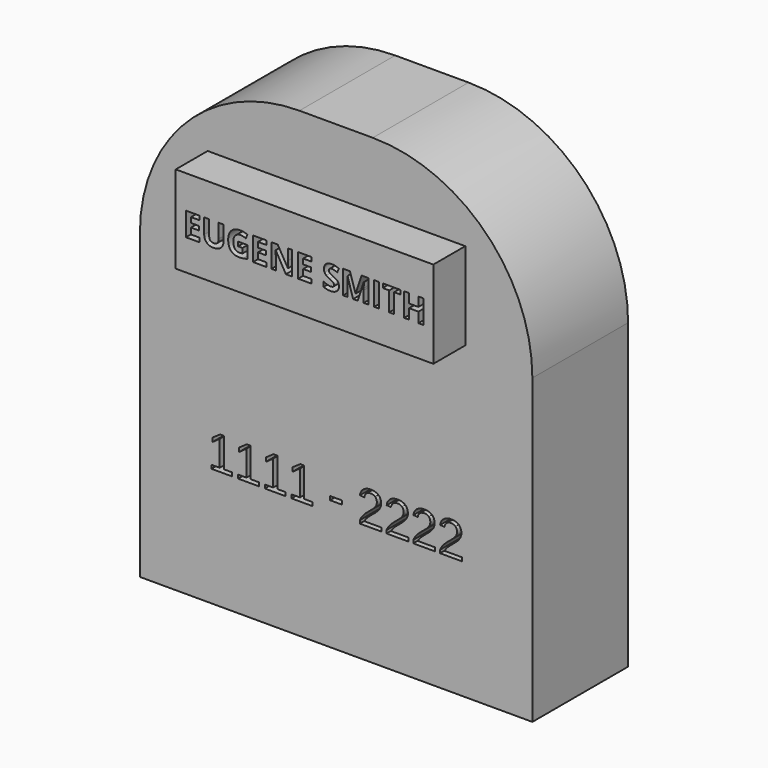
from build123d import *

# Parameters (mm, degrees)
F0_W     = 82.0154622197
F0_H     = 27.821501717
F0_W_2   = 1.5845067707
F0_H_2   = 7.4712192315
F1_DEPTH = 50.8
F0_W_3   = 3.7392849731
F0_H_3   = 1.1961884111
F2_DEPTH = 38.1


with BuildPart() as f1:
    # F0 (on Front) → F1 (new body)
    with BuildSketch(Plane.XZ):
        with Locations((-3.3327825367, 42.5519878045)):
            Rectangle(F0_W, F0_H)
        Polygon((-36.7796089812, 39.8028421267), (-36.7796089812, 38.4946838021), (-41.0818146713, 38.4946838021), (-41.0818146713, 45.9659030336), (-36.7796089812, 45.9659030336), (-36.7796089812, 44.6675558964), (-39.4973079006, 44.6675558964), (-39.4973079006, 43.0274523969), (-36.9676567404, 43.0274523969), (-36.9676567404, 41.7291052597), (-39.4973079006, 41.7291052597), (-39.4973079006, 39.8028421267), align=None, mode=Mode.SUBTRACT)
        with BuildLine():
            Line((-30.7195655424, 45.9659030336), (-29.1399643655, 45.9659030336))
            Line((-29.1399643655, 45.9659030336), (-29.1399643655, 41.1322580241))
            add(Edge.make_bspline(
                [(-29.1399643655, 41.1322580241), (-29.1399643655, 40.3032126859), (-29.5103366911, 39.6802022838)],
                knots=[0, 0, 0, 1, 1, 1], degree=2))
            add(Edge.make_bspline(
                [(-29.5103366911, 39.6802022838), (-29.8807090168, 39.0571918817), (-30.5813913194, 38.7244291079)],
                knots=[0, 0, 0, 1, 1, 1], degree=2))
            add(Edge.make_bspline(
                [(-30.5813913194, 38.7244291079), (-31.282073622, 38.3916663341), (-32.237029199, 38.3916663341)],
                knots=[0, 0, 0, 1, 1, 1], degree=2))
            add(Edge.make_bspline(
                [(-32.237029199, 38.3916663341), (-33.677638554, 38.3916663341), (-34.474797533, 39.1307757875)],
                knots=[0, 0, 0, 1, 1, 1], degree=2))
            add(Edge.make_bspline(
                [(-34.474797533, 39.1307757875), (-35.2719565121, 39.8698852409), (-35.2719565121, 41.151880399)],
                knots=[0, 0, 0, 1, 1, 1], degree=2))
            Line((-35.2719565121, 41.151880399), (-35.2719565121, 45.9659030336))
            Line((-35.2719565121, 45.9659030336), (-33.693990533, 45.9659030336))
            Line((-33.693990533, 45.9659030336), (-33.693990533, 41.3922544912))
            add(Edge.make_bspline(
                [(-33.693990533, 41.3922544912), (-33.693990533, 40.5288699969), (-33.3465109781, 40.1249761142)],
                knots=[0, 0, 0, 1, 1, 1], degree=2))
            add(Edge.make_bspline(
                [(-33.3465109781, 40.1249761142), (-32.9990314231, 39.7210822315), (-32.1961492513, 39.7210822315)],
                knots=[0, 0, 0, 1, 1, 1], degree=2))
            add(Edge.make_bspline(
                [(-32.1961492513, 39.7210822315), (-31.4194302461, 39.7210822315), (-31.0694978943, 40.127428911)],
                knots=[0, 0, 0, 1, 1, 1], degree=2))
            add(Edge.make_bspline(
                [(-31.0694978943, 40.127428911), (-30.7195655424, 40.5337755906), (-30.7195655424, 41.4020656786)],
                knots=[0, 0, 0, 1, 1, 1], degree=2))
            Line((-30.7195655424, 41.4020656786), (-30.7195655424, 45.9659030336))
        make_face(mode=Mode.SUBTRACT)
        with BuildLine():
            Line((-24.4747447403, 41.3709969184), (-24.4747447403, 42.6906016283))
            Line((-24.4747447403, 42.6906016283), (-21.5101309371, 42.6906016283))
            Line((-21.5101309371, 42.6906016283), (-21.5101309371, 38.8168177896))
            add(Edge.make_bspline(
                [(-21.5101309371, 38.8168177896), (-22.2312532136, 38.5813492911), (-22.8673451989, 38.4865078126)],
                knots=[0, 0, 0, 1, 1, 1], degree=2))
            add(Edge.make_bspline(
                [(-22.8673451989, 38.4865078126), (-23.5034371843, 38.3916663341), (-24.167327534, 38.3916663341)],
                knots=[0, 0, 0, 1, 1, 1], degree=2))
            add(Edge.make_bspline(
                [(-24.167327534, 38.3916663341), (-25.8581221686, 38.3916663341), (-26.7501226262, 39.3858666608)],
                knots=[0, 0, 0, 1, 1, 1], degree=2))
            add(Edge.make_bspline(
                [(-26.7501226262, 39.3858666608), (-27.6421230838, 40.3800669875), (-27.6421230838, 42.2409222043)],
                knots=[0, 0, 0, 1, 1, 1], degree=2))
            add(Edge.make_bspline(
                [(-27.6421230838, 42.2409222043), (-27.6421230838, 44.049451088), (-26.6070428094, 45.0608209928)],
                knots=[0, 0, 0, 1, 1, 1], degree=2))
            add(Edge.make_bspline(
                [(-26.6070428094, 45.0608209928), (-25.5719625351, 46.0721908975), (-23.7389056827, 46.0721908975)],
                knots=[0, 0, 0, 1, 1, 1], degree=2))
            add(Edge.make_bspline(
                [(-23.7389056827, 46.0721908975), (-22.587726357, 46.0721908975), (-21.5199421246, 45.612700286)],
                knots=[0, 0, 0, 1, 1, 1], degree=2))
            Line((-21.5199421246, 45.612700286), (-22.0464758502, 44.345421909))
            add(Edge.make_bspline(
                [(-22.0464758502, 44.345421909), (-22.8640748031, 44.7542213854), (-23.7487168701, 44.7542213854)],
                knots=[0, 0, 0, 1, 1, 1], degree=2))
            add(Edge.make_bspline(
                [(-23.7487168701, 44.7542213854), (-24.7756211549, 44.7542213854), (-25.3937259633, 44.0641678692)],
                knots=[0, 0, 0, 1, 1, 1], degree=2))
            add(Edge.make_bspline(
                [(-25.3937259633, 44.0641678692), (-26.0118307717, 43.374114353), (-26.0118307717, 42.209853444)],
                knots=[0, 0, 0, 1, 1, 1], degree=2))
            add(Edge.make_bspline(
                [(-26.0118307717, 42.209853444), (-26.0118307717, 40.9932662021), (-25.5139130094, 40.3522686231)],
                knots=[0, 0, 0, 1, 1, 1], degree=2))
            add(Edge.make_bspline(
                [(-25.5139130094, 40.3522686231), (-25.0159952471, 39.711271044), (-24.0659452638, 39.711271044)],
                knots=[0, 0, 0, 1, 1, 1], degree=2))
            add(Edge.make_bspline(
                [(-24.0659452638, 39.711271044), (-23.5688451005, 39.711271044), (-23.0586633539, 39.8126533142)],
                knots=[0, 0, 0, 1, 1, 1], degree=2))
            Line((-23.0586633539, 39.8126533142), (-23.0586633539, 41.3709969184))
            Line((-23.0586633539, 41.3709969184), (-24.4747447403, 41.3709969184))
        make_face(mode=Mode.SUBTRACT)
        Polygon((-15.4304651235, 39.8028421267), (-15.4304651235, 38.4946838021), (-19.7326708135, 38.4946838021), (-19.7326708135, 45.9659030336), (-15.4304651235, 45.9659030336), (-15.4304651235, 44.6675558964), (-18.1481640429, 44.6675558964), (-18.1481640429, 43.0274523969), (-15.6185128826, 43.0274523969), (-15.6185128826, 41.7291052597), (-18.1481640429, 41.7291052597), (-18.1481640429, 39.8028421267), align=None, mode=Mode.SUBTRACT)
        with BuildLine():
            Line((-7.2446644072, 45.9659030336), (-7.2446644072, 38.4946838021))
            Line((-7.2446644072, 38.4946838021), (-9.2575930292, 38.4946838021))
            Line((-9.2575930292, 38.4946838021), (-12.5083664658, 44.1459277645))
            Line((-12.5083664658, 44.1459277645), (-12.5541520072, 44.1459277645))
            add(Edge.make_bspline(
                [(-12.5541520072, 44.1459277645), (-12.4560401329, 42.6497216807), (-12.4560401329, 42.0103592995)],
                knots=[0, 0, 0, 1, 1, 1], degree=2))
            Line((-12.4560401329, 42.0103592995), (-12.4560401329, 38.4946838021))
            Line((-12.4560401329, 38.4946838021), (-13.8721215193, 38.4946838021))
            Line((-13.8721215193, 38.4946838021), (-13.8721215193, 45.9659030336))
            Line((-13.8721215193, 45.9659030336), (-11.8739096784, 45.9659030336))
            Line((-11.8739096784, 45.9659030336), (-8.6296770334, 40.3702558))
            Line((-8.6296770334, 40.3702558), (-8.5937026794, 40.3702558))
            add(Edge.make_bspline(
                [(-8.5937026794, 40.3702558), (-8.670556981, 41.8272171341), (-8.670556981, 42.4289699634)],
                knots=[0, 0, 0, 1, 1, 1], degree=2))
            Line((-8.670556981, 42.4289699634), (-8.670556981, 45.9659030336))
            Line((-8.670556981, 45.9659030336), (-7.2446644072, 45.9659030336))
        make_face(mode=Mode.SUBTRACT)
        Polygon((-1.0619811254, 39.8028421267), (-1.0619811254, 38.4946838021), (-5.3641868155, 38.4946838021), (-5.3641868155, 45.9659030336), (-1.0619811254, 45.9659030336), (-1.0619811254, 44.6675558964), (-3.7796800448, 44.6675558964), (-3.7796800448, 43.0274523969), (-1.2500288846, 43.0274523969), (-1.2500288846, 41.7291052597), (-3.7796800448, 41.7291052597), (-3.7796800448, 39.8028421267), align=None, mode=Mode.SUBTRACT)
        with BuildLine():
            add(Edge.make_bspline(
                [(7.2374658453, 41.8035067645), (7.6258253479, 41.3006834084), (7.6258253479, 40.5697499446)],
                knots=[0, 0, 0, 1, 1, 1], degree=2))
            add(Edge.make_bspline(
                [(7.6258253479, 40.5697499446), (7.6258253479, 39.5575624409), (6.8973446809, 38.9746143875)],
                knots=[0, 0, 0, 1, 1, 1], degree=2))
            add(Edge.make_bspline(
                [(6.8973446809, 38.9746143875), (6.1688640139, 38.3916663341), (4.8721520746, 38.3916663341)],
                knots=[0, 0, 0, 1, 1, 1], degree=2))
            add(Edge.make_bspline(
                [(4.8721520746, 38.3916663341), (3.6751872076, 38.3916663341), (2.7562059845, 38.8429809561)],
                knots=[0, 0, 0, 1, 1, 1], degree=2))
            Line((2.7562059845, 38.8429809561), (2.7562059845, 40.3146590713))
            add(Edge.make_bspline(
                [(2.7562059845, 40.3146590713), (3.511667417, 39.9761731048), (4.0357483458, 39.8388164807)],
                knots=[0, 0, 0, 1, 1, 1], degree=2))
            add(Edge.make_bspline(
                [(4.0357483458, 39.8388164807), (4.5598292746, 39.7014598566), (4.9947919175, 39.7014598566)],
                knots=[0, 0, 0, 1, 1, 1], degree=2))
            add(Edge.make_bspline(
                [(4.9947919175, 39.7014598566), (5.5147848516, 39.7014598566), (5.7935860945, 39.9001364021)],
                knots=[0, 0, 0, 1, 1, 1], degree=2))
            add(Edge.make_bspline(
                [(5.7935860945, 39.9001364021), (6.0723873374, 40.0988129477), (6.0723873374, 40.492895643)],
                knots=[0, 0, 0, 1, 1, 1], degree=2))
            add(Edge.make_bspline(
                [(6.0723873374, 40.492895643), (6.0723873374, 40.7120121624), (5.9497474945, 40.8837079425)],
                knots=[0, 0, 0, 1, 1, 1], degree=2))
            add(Edge.make_bspline(
                [(5.9497474945, 40.8837079425), (5.8271076516, 41.0554037226), (5.5891863563, 41.2132003205)],
                knots=[0, 0, 0, 1, 1, 1], degree=2))
            add(Edge.make_bspline(
                [(5.5891863563, 41.2132003205), (5.351265061, 41.3709969184), (4.6203315971, 41.7192940723)],
                knots=[0, 0, 0, 1, 1, 1], degree=2))
            add(Edge.make_bspline(
                [(4.6203315971, 41.7192940723), (3.9368188725, 42.0414280597), (3.5942449112, 42.3373988807)],
                knots=[0, 0, 0, 1, 1, 1], degree=2))
            add(Edge.make_bspline(
                [(3.5942449112, 42.3373988807), (3.25167095, 42.6333697016), (3.0472712118, 43.0274523969)],
                knots=[0, 0, 0, 1, 1, 1], degree=2))
            add(Edge.make_bspline(
                [(3.0472712118, 43.0274523969), (2.8428714735, 43.4215350922), (2.8428714735, 43.94643362)],
                knots=[0, 0, 0, 1, 1, 1], degree=2))
            add(Edge.make_bspline(
                [(2.8428714735, 43.94643362), (2.8428714735, 44.9389987488), (3.5149378128, 45.5055948231)],
                knots=[0, 0, 0, 1, 1, 1], degree=2))
            add(Edge.make_bspline(
                [(3.5149378128, 45.5055948231), (4.1870041521, 46.0721908975), (5.3725226338, 46.0721908975)],
                knots=[0, 0, 0, 1, 1, 1], degree=2))
            add(Edge.make_bspline(
                [(5.3725226338, 46.0721908975), (5.9546530882, 46.0721908975), (6.4836396107, 45.9348342734)],
                knots=[0, 0, 0, 1, 1, 1], degree=2))
            add(Edge.make_bspline(
                [(6.4836396107, 45.9348342734), (7.0126261333, 45.7974776493), (7.589850994, 45.5472923697)],
                knots=[0, 0, 0, 1, 1, 1], degree=2))
            Line((7.589850994, 45.5472923697), (7.0796692474, 44.3143531488))
            add(Edge.make_bspline(
                [(7.0796692474, 44.3143531488), (6.4811868139, 44.5596328346), (6.0903745144, 44.65692711)],
                knots=[0, 0, 0, 1, 1, 1], degree=2))
            add(Edge.make_bspline(
                [(6.0903745144, 44.65692711), (5.6995622149, 44.7542213854), (5.3218314987, 44.7542213854)],
                knots=[0, 0, 0, 1, 1, 1], degree=2))
            add(Edge.make_bspline(
                [(5.3218314987, 44.7542213854), (4.8721520746, 44.7542213854), (4.6317779825, 44.5449160535)],
                knots=[0, 0, 0, 1, 1, 1], degree=2))
            add(Edge.make_bspline(
                [(4.6317779825, 44.5449160535), (4.3914038903, 44.3356107215), (4.3914038903, 43.998759953)],
                knots=[0, 0, 0, 1, 1, 1], degree=2))
            add(Edge.make_bspline(
                [(4.3914038903, 43.998759953), (4.3914038903, 43.789454621), (4.4886981657, 43.633293221)],
                knots=[0, 0, 0, 1, 1, 1], degree=2))
            add(Edge.make_bspline(
                [(4.4886981657, 43.633293221), (4.5859924411, 43.477131821), (4.7977505699, 43.3315992074)],
                knots=[0, 0, 0, 1, 1, 1], degree=2))
            add(Edge.make_bspline(
                [(4.7977505699, 43.3315992074), (5.0095086987, 43.1860665938), (5.8009444851, 42.8083358776)],
                knots=[0, 0, 0, 1, 1, 1], degree=2))
            add(Edge.make_bspline(
                [(5.8009444851, 42.8083358776), (6.8491063427, 42.3063301205), (7.2374658453, 41.8035067645)],
                knots=[0, 0, 0, 1, 1, 1], degree=2))
        make_face(mode=Mode.SUBTRACT)
        with BuildLine():
            Line((13.594297704, 38.4946838021), (12.1422419637, 38.4946838021))
            Line((12.1422419637, 38.4946838021), (10.3435242673, 44.3552330964))
            Line((10.3435242673, 44.3552330964), (10.297738726, 44.3552330964))
            add(Edge.make_bspline(
                [(10.297738726, 44.3552330964), (10.3958506003, 42.5679617854), (10.3958506003, 41.9694793519)],
                knots=[0, 0, 0, 1, 1, 1], degree=2))
            Line((10.3958506003, 41.9694793519), (10.3958506003, 38.4946838021))
            Line((10.3958506003, 38.4946838021), (8.9797692139, 38.4946838021))
            Line((8.9797692139, 38.4946838021), (8.9797692139, 45.9659030336))
            Line((8.9797692139, 45.9659030336), (11.1365952516, 45.9659030336))
            Line((11.1365952516, 45.9659030336), (12.9042441878, 40.2525215508))
            Line((12.9042441878, 40.2525215508), (12.935312948, 40.2525215508))
            Line((12.935312948, 40.2525215508), (14.8108849459, 45.9659030336))
            Line((14.8108849459, 45.9659030336), (16.9660757857, 45.9659030336))
            Line((16.9660757857, 45.9659030336), (16.9660757857, 38.4946838021))
            Line((16.9660757857, 38.4946838021), (15.4894920768, 38.4946838021))
            Line((15.4894920768, 38.4946838021), (15.4894920768, 42.0316168723))
            add(Edge.make_bspline(
                [(15.4894920768, 42.0316168723), (15.4894920768, 42.2818021519), (15.4976680663, 42.608841733)],
                knots=[0, 0, 0, 1, 1, 1], degree=2))
            add(Edge.make_bspline(
                [(15.4976680663, 42.608841733), (15.5058440558, 42.9358813142), (15.5663463783, 44.345421909)],
                knots=[0, 0, 0, 1, 1, 1], degree=2))
            Line((15.5663463783, 44.345421909), (15.520560837, 44.345421909))
            Line((15.520560837, 44.345421909), (13.594297704, 38.4946838021))
        make_face(mode=Mode.SUBTRACT)
        with Locations((19.6388067627, 42.2302934179)):
            Rectangle(F0_W_2, F0_H_2, mode=Mode.SUBTRACT)
        Polygon((25.1943916475, 44.6479335215), (25.1943916475, 38.4946838021), (23.6098848768, 38.4946838021), (23.6098848768, 44.6479335215), (21.5806042758, 44.6479335215), (21.5806042758, 45.9659030336), (27.2220370507, 45.9659030336), (27.2220370507, 44.6479335215), align=None, mode=Mode.SUBTRACT)
        Polygon((34.4937621377, 45.9659030336), (34.4937621377, 38.4946838021), (32.9141609607, 38.4946838021), (32.9141609607, 41.7192940723), (29.9560879491, 41.7192940723), (29.9560879491, 38.4946838021), (28.3715811784, 38.4946838021), (28.3715811784, 45.9659030336), (29.9560879491, 45.9659030336), (29.9560879491, 43.0372635844), (32.9141609607, 43.0372635844), (32.9141609607, 45.9659030336), align=None, mode=Mode.SUBTRACT)
    extrude(amount=F1_DEPTH)

    # F0 (on Front) → F2 (join)
    with BuildSketch(Plane.XZ):
        with BuildLine():
            Line((-65.9075155854, 26.4598572791), (-65.9075155854, -69.9368044734))
            Line((-65.9075155854, -69.9368044734), (59.0424365504, -69.9368044734))
            Line((59.0424365504, -69.9368044734), (59.0424365504, 26.4598572791))
            ThreePointArc((59.0424365504, 26.4598572791), (44.1634610346, 62.3808817633), (8.2424365504, 77.2598572791))
            Line((8.2424365504, 77.2598572791), (-15.1075155854, 77.2598572791))
            ThreePointArc((-15.1075155854, 77.2598572791), (-51.0285400697, 62.3808817633), (-65.9075155854, 26.4598572791))
        make_face()
        Polygon((-36.5724661048, -32.2220926494), (-43.1730337574, -32.2220926494), (-43.1730337574, -31.0785365283), (-40.4911793396, -31.0785365283), (-40.4911793396, -22.9731638546), (-42.8668095241, -24.6717513984), (-42.8668095241, -23.399006929), (-40.378737629, -21.6884575011), (-39.1370940583, -21.6884575011), (-39.1370940583, -31.0785365283), (-36.5724661048, -31.0785365283), align=None, mode=Mode.SUBTRACT)
        Polygon((-28.0579969945, -32.2220926494), (-34.658564647, -32.2220926494), (-34.658564647, -31.0785365283), (-31.9767102293, -31.0785365283), (-31.9767102293, -22.9731638546), (-34.3523404138, -24.6717513984), (-34.3523404138, -23.399006929), (-31.8642685187, -21.6884575011), (-30.6226249479, -21.6884575011), (-30.6226249479, -31.0785365283), (-28.0579969945, -31.0785365283), align=None, mode=Mode.SUBTRACT)
        Polygon((-19.5435278842, -32.2220926494), (-26.1440955367, -32.2220926494), (-26.1440955367, -31.0785365283), (-23.462241119, -31.0785365283), (-23.462241119, -22.9731638546), (-25.8378713035, -24.6717513984), (-25.8378713035, -23.399006929), (-23.3497994083, -21.6884575011), (-22.1081558376, -21.6884575011), (-22.1081558376, -31.0785365283), (-19.5435278842, -31.0785365283), align=None, mode=Mode.SUBTRACT)
        Polygon((-11.0290587739, -32.2220926494), (-17.6296264264, -32.2220926494), (-17.6296264264, -31.0785365283), (-14.9477720087, -31.0785365283), (-14.9477720087, -22.9731638546), (-17.3234021932, -24.6717513984), (-17.3234021932, -23.399006929), (-14.835330298, -21.6884575011), (-13.5936867273, -21.6884575011), (-13.5936867273, -31.0785365283), (-11.0290587739, -31.0785365283), align=None, mode=Mode.SUBTRACT)
        with Locations((-3.4799137113, -28.1550520516)):
            Rectangle(F0_W_3, F0_H_3, mode=Mode.SUBTRACT)
        with BuildLine():
            Line((11.0693259331, -32.2220926494), (4.0931551195, -32.2220926494))
            Line((4.0931551195, -32.2220926494), (4.0931551195, -31.2723190509))
            add(Edge.make_bspline(
                [(4.0931551195, -31.2723190509), (4.4735430342, -30.396709134), (5.0237897033, -29.7280398122)],
                knots=[0, 0, 0, 1, 1, 1], degree=2))
            add(Edge.make_bspline(
                [(5.0237897033, -29.7280398122), (5.5740363724, -29.0593704904), (6.1793077084, -28.5174971401)],
                knots=[0, 0, 0, 1, 1, 1], degree=2))
            add(Edge.make_bspline(
                [(6.1793077084, -28.5174971401), (6.7845790445, -27.9756237899), (7.3790846848, -27.5115026864)],
                knots=[0, 0, 0, 1, 1, 1], degree=2))
            add(Edge.make_bspline(
                [(7.3790846848, -27.5115026864), (7.9735903251, -27.0473815829), (8.4520656896, -26.5844566678)],
                knots=[0, 0, 0, 1, 1, 1], degree=2))
            add(Edge.make_bspline(
                [(8.4520656896, -26.5844566678), (8.930541054, -26.1215317527), (9.2259995916, -25.613151678)],
                knots=[0, 0, 0, 1, 1, 1], degree=2))
            add(Edge.make_bspline(
                [(9.2259995916, -25.613151678), (9.5214581291, -25.1047716032), (9.5214581291, -24.4612222381)],
                knots=[0, 0, 0, 1, 1, 1], degree=2))
            add(Edge.make_bspline(
                [(9.5214581291, -24.4612222381), (9.5214581291, -23.5951818284), (9.0130780544, -23.116706464)],
                knots=[0, 0, 0, 1, 1, 1], degree=2))
            add(Edge.make_bspline(
                [(9.0130780544, -23.116706464), (8.5046979797, -22.6382310995), (7.6003795408, -22.6382310995)],
                knots=[0, 0, 0, 1, 1, 1], degree=2))
            add(Edge.make_bspline(
                [(7.6003795408, -22.6382310995), (6.7391238848, -22.6382310995), (6.1828962737, -23.1047445798)],
                knots=[0, 0, 0, 1, 1, 1], degree=2))
            add(Edge.make_bspline(
                [(6.1828962737, -23.1047445798), (5.6266686625, -23.5712580602), (5.5285812128, -24.4157670784)],
                knots=[0, 0, 0, 1, 1, 1], degree=2))
            Line((5.5285812128, -24.4157670784), (4.15296454, -24.2889711069))
            add(Edge.make_bspline(
                [(4.15296454, -24.2889711069), (4.301291903, -23.0257961447), (5.2247493564, -22.2781783878)],
                knots=[0, 0, 0, 1, 1, 1], degree=2))
            add(Edge.make_bspline(
                [(5.2247493564, -22.2781783878), (6.1482068098, -21.5305606308), (7.6003795408, -21.5305606308)],
                knots=[0, 0, 0, 1, 1, 1], degree=2))
            add(Edge.make_bspline(
                [(7.6003795408, -21.5305606308), (9.1913101276, -21.5305606308), (10.04778103, -22.281766953)],
                knots=[0, 0, 0, 1, 1, 1], degree=2))
            add(Edge.make_bspline(
                [(10.04778103, -22.281766953), (10.9042519324, -23.0329732752), (10.9042519324, -24.4157670784)],
                knots=[0, 0, 0, 1, 1, 1], degree=2))
            add(Edge.make_bspline(
                [(10.9042519324, -24.4157670784), (10.9042519324, -25.0306079217), (10.6231476557, -25.6358792578)],
                knots=[0, 0, 0, 1, 1, 1], degree=2))
            add(Edge.make_bspline(
                [(10.6231476557, -25.6358792578), (10.3420433791, -26.2411505938), (9.7894043332, -26.8464219298)],
                knots=[0, 0, 0, 1, 1, 1], degree=2))
            add(Edge.make_bspline(
                [(9.7894043332, -26.8464219298), (9.2367652873, -27.4516932658), (7.6745432223, -28.7220453584)],
                knots=[0, 0, 0, 1, 1, 1], degree=2))
            add(Edge.make_bspline(
                [(7.6745432223, -28.7220453584), (6.8132875663, -29.4254041442), (6.3049074916, -29.9900050742)],
                knots=[0, 0, 0, 1, 1, 1], degree=2))
            add(Edge.make_bspline(
                [(6.3049074916, -29.9900050742), (5.7965274169, -30.5546060043), (5.5740363724, -31.0785365283)],
                knots=[0, 0, 0, 1, 1, 1], degree=2))
            Line((5.5740363724, -31.0785365283), (11.0693259331, -31.0785365283))
            Line((11.0693259331, -31.0785365283), (11.0693259331, -32.2220926494))
        make_face(mode=Mode.SUBTRACT)
        with BuildLine():
            Line((19.5837950434, -32.2220926494), (12.6076242298, -32.2220926494))
            Line((12.6076242298, -32.2220926494), (12.6076242298, -31.2723190509))
            add(Edge.make_bspline(
                [(12.6076242298, -31.2723190509), (12.9880121445, -30.396709134), (13.5382588136, -29.7280398122)],
                knots=[0, 0, 0, 1, 1, 1], degree=2))
            add(Edge.make_bspline(
                [(13.5382588136, -29.7280398122), (14.0885054827, -29.0593704904), (14.6937768188, -28.5174971401)],
                knots=[0, 0, 0, 1, 1, 1], degree=2))
            add(Edge.make_bspline(
                [(14.6937768188, -28.5174971401), (15.2990481548, -27.9756237899), (15.8935537951, -27.5115026864)],
                knots=[0, 0, 0, 1, 1, 1], degree=2))
            add(Edge.make_bspline(
                [(15.8935537951, -27.5115026864), (16.4880594354, -27.0473815829), (16.9665347999, -26.5844566678)],
                knots=[0, 0, 0, 1, 1, 1], degree=2))
            add(Edge.make_bspline(
                [(16.9665347999, -26.5844566678), (17.4450101643, -26.1215317527), (17.7404687019, -25.613151678)],
                knots=[0, 0, 0, 1, 1, 1], degree=2))
            add(Edge.make_bspline(
                [(17.7404687019, -25.613151678), (18.0359272394, -25.1047716032), (18.0359272394, -24.4612222381)],
                knots=[0, 0, 0, 1, 1, 1], degree=2))
            add(Edge.make_bspline(
                [(18.0359272394, -24.4612222381), (18.0359272394, -23.5951818284), (17.5275471647, -23.116706464)],
                knots=[0, 0, 0, 1, 1, 1], degree=2))
            add(Edge.make_bspline(
                [(17.5275471647, -23.116706464), (17.01916709, -22.6382310995), (16.1148486512, -22.6382310995)],
                knots=[0, 0, 0, 1, 1, 1], degree=2))
            add(Edge.make_bspline(
                [(16.1148486512, -22.6382310995), (15.2535929952, -22.6382310995), (14.697365384, -23.1047445798)],
                knots=[0, 0, 0, 1, 1, 1], degree=2))
            add(Edge.make_bspline(
                [(14.697365384, -23.1047445798), (14.1411377728, -23.5712580602), (14.0430503231, -24.4157670784)],
                knots=[0, 0, 0, 1, 1, 1], degree=2))
            Line((14.0430503231, -24.4157670784), (12.6674336503, -24.2889711069))
            add(Edge.make_bspline(
                [(12.6674336503, -24.2889711069), (12.8157610133, -23.0257961447), (13.7392184667, -22.2781783878)],
                knots=[0, 0, 0, 1, 1, 1], degree=2))
            add(Edge.make_bspline(
                [(13.7392184667, -22.2781783878), (14.6626759201, -21.5305606308), (16.1148486512, -21.5305606308)],
                knots=[0, 0, 0, 1, 1, 1], degree=2))
            add(Edge.make_bspline(
                [(16.1148486512, -21.5305606308), (17.705779238, -21.5305606308), (18.5622501403, -22.281766953)],
                knots=[0, 0, 0, 1, 1, 1], degree=2))
            add(Edge.make_bspline(
                [(18.5622501403, -22.281766953), (19.4187210427, -23.0329732752), (19.4187210427, -24.4157670784)],
                knots=[0, 0, 0, 1, 1, 1], degree=2))
            add(Edge.make_bspline(
                [(19.4187210427, -24.4157670784), (19.4187210427, -25.0306079217), (19.1376167661, -25.6358792578)],
                knots=[0, 0, 0, 1, 1, 1], degree=2))
            add(Edge.make_bspline(
                [(19.1376167661, -25.6358792578), (18.8565124894, -26.2411505938), (18.3038734435, -26.8464219298)],
                knots=[0, 0, 0, 1, 1, 1], degree=2))
            add(Edge.make_bspline(
                [(18.3038734435, -26.8464219298), (17.7512343976, -27.4516932658), (16.1890123327, -28.7220453584)],
                knots=[0, 0, 0, 1, 1, 1], degree=2))
            add(Edge.make_bspline(
                [(16.1890123327, -28.7220453584), (15.3277566767, -29.4254041442), (14.8193766019, -29.9900050742)],
                knots=[0, 0, 0, 1, 1, 1], degree=2))
            add(Edge.make_bspline(
                [(14.8193766019, -29.9900050742), (14.3109965272, -30.5546060043), (14.0885054827, -31.0785365283)],
                knots=[0, 0, 0, 1, 1, 1], degree=2))
            Line((14.0885054827, -31.0785365283), (19.5837950434, -31.0785365283))
            Line((19.5837950434, -31.0785365283), (19.5837950434, -32.2220926494))
        make_face(mode=Mode.SUBTRACT)
        with BuildLine():
            Line((28.0982641537, -32.2220926494), (21.1220933401, -32.2220926494))
            Line((21.1220933401, -32.2220926494), (21.1220933401, -31.2723190509))
            add(Edge.make_bspline(
                [(21.1220933401, -31.2723190509), (21.5024812548, -30.396709134), (22.0527279239, -29.7280398122)],
                knots=[0, 0, 0, 1, 1, 1], degree=2))
            add(Edge.make_bspline(
                [(22.0527279239, -29.7280398122), (22.6029745931, -29.0593704904), (23.2082459291, -28.5174971401)],
                knots=[0, 0, 0, 1, 1, 1], degree=2))
            add(Edge.make_bspline(
                [(23.2082459291, -28.5174971401), (23.8135172651, -27.9756237899), (24.4080229054, -27.5115026864)],
                knots=[0, 0, 0, 1, 1, 1], degree=2))
            add(Edge.make_bspline(
                [(24.4080229054, -27.5115026864), (25.0025285458, -27.0473815829), (25.4810039102, -26.5844566678)],
                knots=[0, 0, 0, 1, 1, 1], degree=2))
            add(Edge.make_bspline(
                [(25.4810039102, -26.5844566678), (25.9594792746, -26.1215317527), (26.2549378122, -25.613151678)],
                knots=[0, 0, 0, 1, 1, 1], degree=2))
            add(Edge.make_bspline(
                [(26.2549378122, -25.613151678), (26.5503963497, -25.1047716032), (26.5503963497, -24.4612222381)],
                knots=[0, 0, 0, 1, 1, 1], degree=2))
            add(Edge.make_bspline(
                [(26.5503963497, -24.4612222381), (26.5503963497, -23.5951818284), (26.042016275, -23.116706464)],
                knots=[0, 0, 0, 1, 1, 1], degree=2))
            add(Edge.make_bspline(
                [(26.042016275, -23.116706464), (25.5336362003, -22.6382310995), (24.6293177615, -22.6382310995)],
                knots=[0, 0, 0, 1, 1, 1], degree=2))
            add(Edge.make_bspline(
                [(24.6293177615, -22.6382310995), (23.7680621055, -22.6382310995), (23.2118344943, -23.1047445798)],
                knots=[0, 0, 0, 1, 1, 1], degree=2))
            add(Edge.make_bspline(
                [(23.2118344943, -23.1047445798), (22.6556068831, -23.5712580602), (22.5575194334, -24.4157670784)],
                knots=[0, 0, 0, 1, 1, 1], degree=2))
            Line((22.5575194334, -24.4157670784), (21.1819027607, -24.2889711069))
            add(Edge.make_bspline(
                [(21.1819027607, -24.2889711069), (21.3302301236, -23.0257961447), (22.253687577, -22.2781783878)],
                knots=[0, 0, 0, 1, 1, 1], degree=2))
            add(Edge.make_bspline(
                [(22.253687577, -22.2781783878), (23.1771450304, -21.5305606308), (24.6293177615, -21.5305606308)],
                knots=[0, 0, 0, 1, 1, 1], degree=2))
            add(Edge.make_bspline(
                [(24.6293177615, -21.5305606308), (26.2202483483, -21.5305606308), (27.0767192506, -22.281766953)],
                knots=[0, 0, 0, 1, 1, 1], degree=2))
            add(Edge.make_bspline(
                [(27.0767192506, -22.281766953), (27.933190153, -23.0329732752), (27.933190153, -24.4157670784)],
                knots=[0, 0, 0, 1, 1, 1], degree=2))
            add(Edge.make_bspline(
                [(27.933190153, -24.4157670784), (27.933190153, -25.0306079217), (27.6520858764, -25.6358792578)],
                knots=[0, 0, 0, 1, 1, 1], degree=2))
            add(Edge.make_bspline(
                [(27.6520858764, -25.6358792578), (27.3709815998, -26.2411505938), (26.8183425538, -26.8464219298)],
                knots=[0, 0, 0, 1, 1, 1], degree=2))
            add(Edge.make_bspline(
                [(26.8183425538, -26.8464219298), (26.2657035079, -27.4516932658), (24.703481443, -28.7220453584)],
                knots=[0, 0, 0, 1, 1, 1], degree=2))
            add(Edge.make_bspline(
                [(24.703481443, -28.7220453584), (23.842225787, -29.4254041442), (23.3338457123, -29.9900050742)],
                knots=[0, 0, 0, 1, 1, 1], degree=2))
            add(Edge.make_bspline(
                [(23.3338457123, -29.9900050742), (22.8254656375, -30.5546060043), (22.6029745931, -31.0785365283)],
                knots=[0, 0, 0, 1, 1, 1], degree=2))
            Line((22.6029745931, -31.0785365283), (28.0982641537, -31.0785365283))
            Line((28.0982641537, -31.0785365283), (28.0982641537, -32.2220926494))
        make_face(mode=Mode.SUBTRACT)
        with BuildLine():
            Line((36.612733264, -32.2220926494), (29.6365624504, -32.2220926494))
            Line((29.6365624504, -32.2220926494), (29.6365624504, -31.2723190509))
            add(Edge.make_bspline(
                [(29.6365624504, -31.2723190509), (30.0169503652, -30.396709134), (30.5671970343, -29.7280398122)],
                knots=[0, 0, 0, 1, 1, 1], degree=2))
            add(Edge.make_bspline(
                [(30.5671970343, -29.7280398122), (31.1174437034, -29.0593704904), (31.7227150394, -28.5174971401)],
                knots=[0, 0, 0, 1, 1, 1], degree=2))
            add(Edge.make_bspline(
                [(31.7227150394, -28.5174971401), (32.3279863754, -27.9756237899), (32.9224920158, -27.5115026864)],
                knots=[0, 0, 0, 1, 1, 1], degree=2))
            add(Edge.make_bspline(
                [(32.9224920158, -27.5115026864), (33.5169976561, -27.0473815829), (33.9954730205, -26.5844566678)],
                knots=[0, 0, 0, 1, 1, 1], degree=2))
            add(Edge.make_bspline(
                [(33.9954730205, -26.5844566678), (34.473948385, -26.1215317527), (34.7694069225, -25.613151678)],
                knots=[0, 0, 0, 1, 1, 1], degree=2))
            add(Edge.make_bspline(
                [(34.7694069225, -25.613151678), (35.0648654601, -25.1047716032), (35.0648654601, -24.4612222381)],
                knots=[0, 0, 0, 1, 1, 1], degree=2))
            add(Edge.make_bspline(
                [(35.0648654601, -24.4612222381), (35.0648654601, -23.5951818284), (34.5564853853, -23.116706464)],
                knots=[0, 0, 0, 1, 1, 1], degree=2))
            add(Edge.make_bspline(
                [(34.5564853853, -23.116706464), (34.0481053106, -22.6382310995), (33.1437868718, -22.6382310995)],
                knots=[0, 0, 0, 1, 1, 1], degree=2))
            add(Edge.make_bspline(
                [(33.1437868718, -22.6382310995), (32.2825312158, -22.6382310995), (31.7263036046, -23.1047445798)],
                knots=[0, 0, 0, 1, 1, 1], degree=2))
            add(Edge.make_bspline(
                [(31.7263036046, -23.1047445798), (31.1700759935, -23.5712580602), (31.0719885438, -24.4157670784)],
                knots=[0, 0, 0, 1, 1, 1], degree=2))
            Line((31.0719885438, -24.4157670784), (29.696371871, -24.2889711069))
            add(Edge.make_bspline(
                [(29.696371871, -24.2889711069), (29.844699234, -23.0257961447), (30.7681566873, -22.2781783878)],
                knots=[0, 0, 0, 1, 1, 1], degree=2))
            add(Edge.make_bspline(
                [(30.7681566873, -22.2781783878), (31.6916141407, -21.5305606308), (33.1437868718, -21.5305606308)],
                knots=[0, 0, 0, 1, 1, 1], degree=2))
            add(Edge.make_bspline(
                [(33.1437868718, -21.5305606308), (34.7347174586, -21.5305606308), (35.5911883609, -22.281766953)],
                knots=[0, 0, 0, 1, 1, 1], degree=2))
            add(Edge.make_bspline(
                [(35.5911883609, -22.281766953), (36.4476592633, -23.0329732752), (36.4476592633, -24.4157670784)],
                knots=[0, 0, 0, 1, 1, 1], degree=2))
            add(Edge.make_bspline(
                [(36.4476592633, -24.4157670784), (36.4476592633, -25.0306079217), (36.1665549867, -25.6358792578)],
                knots=[0, 0, 0, 1, 1, 1], degree=2))
            add(Edge.make_bspline(
                [(36.1665549867, -25.6358792578), (35.8854507101, -26.2411505938), (35.3328116641, -26.8464219298)],
                knots=[0, 0, 0, 1, 1, 1], degree=2))
            add(Edge.make_bspline(
                [(35.3328116641, -26.8464219298), (34.7801726182, -27.4516932658), (33.2179505533, -28.7220453584)],
                knots=[0, 0, 0, 1, 1, 1], degree=2))
            add(Edge.make_bspline(
                [(33.2179505533, -28.7220453584), (32.3566948973, -29.4254041442), (31.8483148226, -29.9900050742)],
                knots=[0, 0, 0, 1, 1, 1], degree=2))
            add(Edge.make_bspline(
                [(31.8483148226, -29.9900050742), (31.3399347478, -30.5546060043), (31.1174437034, -31.0785365283)],
                knots=[0, 0, 0, 1, 1, 1], degree=2))
            Line((31.1174437034, -31.0785365283), (36.612733264, -31.0785365283))
            Line((36.612733264, -31.0785365283), (36.612733264, -32.2220926494))
        make_face(mode=Mode.SUBTRACT)
        with Locations((-3.3327825367, 42.5519878045)):
            Rectangle(F0_W, F0_H, mode=Mode.SUBTRACT)
    extrude(amount=F2_DEPTH)


solid = f1.part
